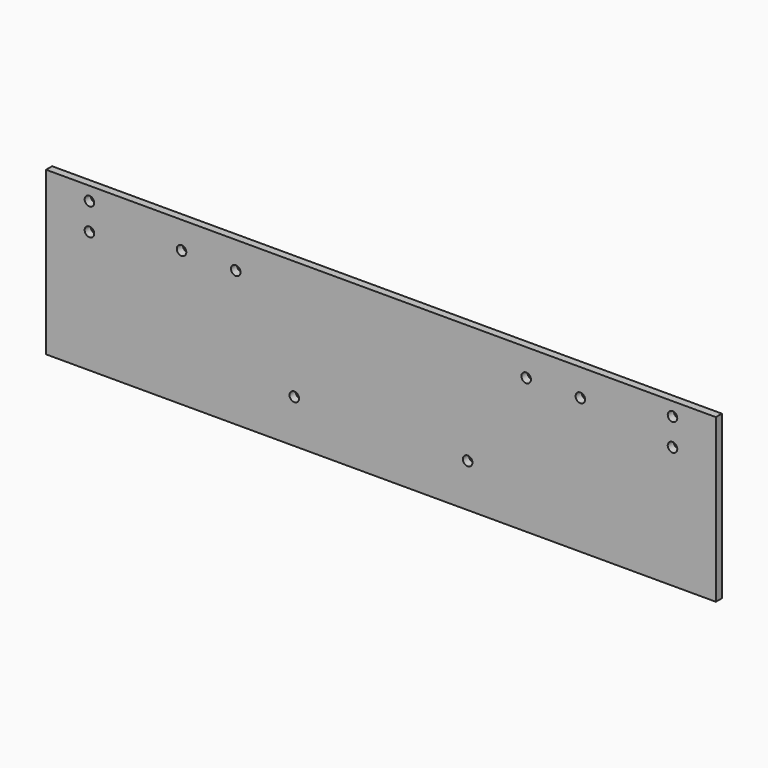
from build123d import *

# Parameters (mm, degrees)
F0_W     = 618
F0_H     = 150
F1_DEPTH = 7
F3_D     = 8.8
F5_D     = 8.8


# Not quite as in the source:
# - a feature names something its author has since deleted; it is built from what else it names


with BuildPart() as f1:
    # F0 (on Front) → F1 (new body)
    with BuildSketch(Plane.XZ):
        with Locations((1, -375)):
            Rectangle(F0_W, F0_H)
    extrude(amount=F1_DEPTH)

    # F3 (through all)
    with Locations(Plane.XZ.offset(7)):
        with Locations((-183, -325), (-133, -325), (185, -325), (135, -325)):
            Hole(F3_D / 2)

    # F5 (through all)
    with Locations(Plane.XZ.offset(7)):
        with Locations((-268, -337.5), (-268, -312.5), (270, -337.5), (270, -312.5), (-79, -410), (81, -410)):
            Hole(F5_D / 2)


solid = f1.part
